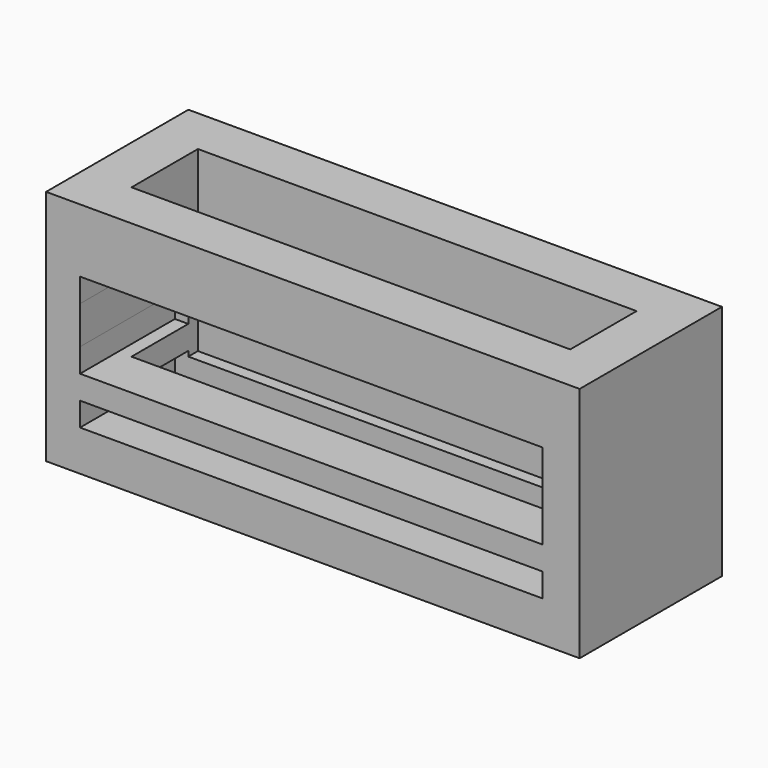
from build123d import *

# Parameters (mm, degrees)
F0_W     = 114.3
F0_H     = 38.1
F1_DEPTH = 50.8
F2_W     = 93.98
F2_H     = 17.78
F3_DEPTH = 38.1
F4_W     = 99.06
F4_H     = 5.08
F5_DEPTH = 25.4
F6_DEPTH = 25.4


# Not quite as in the source:
# - a feature names something its author has since deleted; it is built from what else it names


with BuildPart() as f1:
    # F0 (on Top) → F1 (new body)
    with BuildSketch(Plane.XY):
        with Locations((-0.8744271472, -29.0754930802)):
            Rectangle(F0_W, F0_H)
    extrude(amount=F1_DEPTH)

    # F2 (on face) → F3 (cut)
    with BuildSketch(Plane.XY.offset(50.8)):
        with Locations((-0.8926133716, -29.0383800721)):
            Rectangle(F2_W, F2_H)
    extrude(amount=-F3_DEPTH, mode=Mode.SUBTRACT)

    # F4 (on face) → F5 (cut)
    with BuildSketch(Plane.XZ.offset(48.1254930802)):
        with Locations((-1.2216676867, 11.2467280274)):
            Rectangle(F4_W, F4_H)
        Polygon((-50.7150366902, 32.0992726219), (-50.7516676867, 23.9467280274), (48.3083323133, 23.9467280274), (48.3449633098, 32.0992726219), align=None)
        with Locations((-1.2216676867, 21.4067280274)):
            Rectangle(F4_W, F4_H)
        with Locations((-1.1850366902, 34.6392726219)):
            Rectangle(F4_W, F4_H)
    extrude(amount=-F5_DEPTH, mode=Mode.SUBTRACT)

    # F4 (on face) → F6 (cut)
    with BuildSketch(Plane.XZ.offset(48.1254930802)):
        with Locations((-1.2216676867, 11.2467280274)):
            Rectangle(F4_W, F4_H)
        Polygon((-50.7150366902, 32.0992726219), (-50.7516676867, 23.9467280274), (48.3083323133, 23.9467280274), (48.3449633098, 32.0992726219), align=None)
        with Locations((-1.2216676867, 21.4067280274)):
            Rectangle(F4_W, F4_H)
        with Locations((-1.1850366902, 34.6392726219)):
            Rectangle(F4_W, F4_H)
    extrude(amount=-F6_DEPTH, mode=Mode.SUBTRACT)


solid = f1.part
